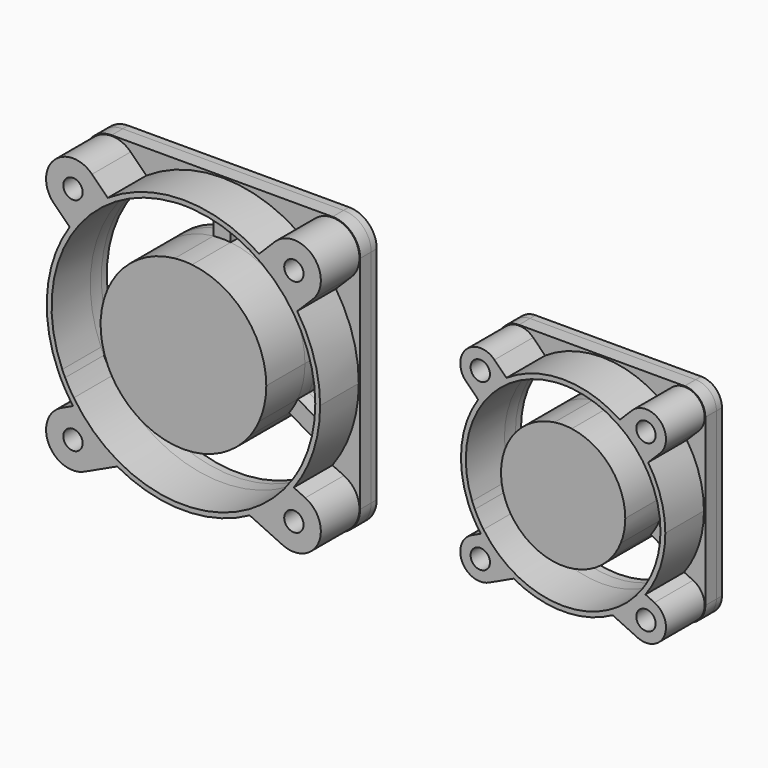
from build123d import *

# Parameters (mm, degrees)
F3_R     = 1.4
F4_DEPTH = 1
F5_DEPTH = 2
F6_DEPTH = 9
F7_DEPTH = 2
F8_DEPTH = 2


with BuildPart() as f4:
    # F3 (on Front) → F4 (new body)
    with BuildSketch(Plane.XZ):
        with BuildLine():
            Line((-16.757716, 18.757716), (-19.031282, 16.484151))
            ThreePointArc((-19.031282, 16.484151), (-15.999286, 14.000714), (-13.515849, 10.968718))
            Line((-13.515849, 10.968718), (-11.242284, 13.242284))
            ThreePointArc((-11.242284, 13.242284), (-11.242284, 18.757716), (-16.757716, 18.757716))
        make_face()
        with Locations((-14, 16)):
            Circle(F3_R, mode=Mode.SUBTRACT)
        with BuildLine():
            ThreePointArc((-45.981912, -11.688391), (-46.921843, -10.280624), (-47.738098, -8.79772))
            Line((-47.738098, -8.79772), (-50, -10.10363))
            Line((-50, -10.10363), (-50, -16))
            ThreePointArc((-50, -16), (-48.828427, -18.828427), (-46, -20))
            Line((-46, -20), (-30, -20))
            Line((-30, -20), (-14, -20))
            ThreePointArc((-14, -20), (-11.171573, -18.828427), (-10, -16))
            Line((-10, -16), (-10, 0))
            Line((-10, 0), (-10, 16))
            ThreePointArc((-10, 16), (-11.171573, 18.828427), (-14, 20))
            Line((-14, 20), (-30, 20))
            Line((-30, 20), (-46, 20))
            ThreePointArc((-46, 20), (-48.828427, 18.828427), (-50, 16))
            Line((-50, 16), (-50, 0))
            Line((-50, 0), (-50, -8.948929))
            Line((-50, -8.948929), (-48.16123, -7.887315))
            ThreePointArc((-48.16123, -7.887315), (-49.722147, 1.754112), (-46.484151, 10.968718))
            Line((-46.484151, 10.968718), (-48.757716, 13.242284))
            ThreePointArc((-48.757716, 13.242284), (-48.757716, 18.757716), (-43.242284, 18.757716))
            Line((-43.242284, 18.757716), (-40.968718, 16.484151))
            ThreePointArc((-40.968718, 16.484151), (-30, 19.8), (-19.031282, 16.484151))
            Line((-19.031282, 16.484151), (-16.757716, 18.757716))
            ThreePointArc((-16.757716, 18.757716), (-11.242284, 18.757716), (-11.242284, 13.242284))
            Line((-11.242284, 13.242284), (-13.515849, 10.968718))
            ThreePointArc((-13.515849, 10.968718), (-11.047082, 5.729477), (-10.2, 0))
            ThreePointArc((-10.2, 0), (-11.178711, -6.148095), (-14.018088, -11.688391))
            Line((-14.018088, -11.688391), (-12.351789, -12.4654))
            ThreePointArc((-12.351789, -12.4654), (-10.4654, -17.648211), (-15.648211, -19.5346))
            Line((-15.648211, -19.5346), (-20.401726, -17.318))
            ThreePointArc((-20.401726, -17.318), (-30, -19.8), (-39.598274, -17.318))
            Line((-39.598274, -17.318), (-44.351789, -19.5346))
            ThreePointArc((-44.351789, -19.5346), (-49.5346, -17.648211), (-47.648211, -12.4654))
            Line((-47.648211, -12.4654), (-45.981912, -11.688391))
        make_face()
        with BuildLine():
            ThreePointArc((-31.25, 19.059053), (-30, 19.1), (-28.75, 19.059053))
            ThreePointArc((-28.75, 19.059053), (-16.059322, 13.05632), (-10.9, 0))
            ThreePointArc((-10.9, 0), (-11.398859, -4.336766), (-12.869376, -8.446995))
            ThreePointArc((-12.869376, -8.446995), (-13.458915, -9.55), (-14.119376, -10.612058))
            ThreePointArc((-14.119376, -10.612058), (-30, -19.1), (-45.880624, -10.612058))
            ThreePointArc((-45.880624, -10.612058), (-46.541085, -9.55), (-47.130624, -8.446995))
            Line((-47.130624, -8.446995), (-47.738098, -8.79772))
            ThreePointArc((-47.738098, -8.79772), (-46.921843, -10.280624), (-45.981912, -11.688391))
            ThreePointArc((-45.981912, -11.688391), (-43.096168, -14.850266), (-39.598274, -17.318))
            ThreePointArc((-39.598274, -17.318), (-30, -19.8), (-20.401726, -17.318))
            ThreePointArc((-20.401726, -17.318), (-16.903832, -14.850266), (-14.018088, -11.688391))
            ThreePointArc((-14.018088, -11.688391), (-11.178711, -6.148095), (-10.2, 0))
            ThreePointArc((-10.2, 0), (-11.047082, 5.729477), (-13.515849, 10.968718))
            ThreePointArc((-13.515849, 10.968718), (-15.999286, 14.000714), (-19.031282, 16.484151))
            ThreePointArc((-19.031282, 16.484151), (-30, 19.8), (-40.968718, 16.484151))
            ThreePointArc((-40.968718, 16.484151), (-44.000714, 14.000714), (-46.484151, 10.968718))
            ThreePointArc((-46.484151, 10.968718), (-49.722147, 1.754112), (-48.16123, -7.887315))
            Line((-48.16123, -7.887315), (-47.550913, -7.534948))
            ThreePointArc((-47.550913, -7.534948), (-46.284312, 9.981542), (-31.25, 19.059053))
        make_face()
        with BuildLine():
            Line((-48.757716, 13.242284), (-46.484151, 10.968718))
            ThreePointArc((-46.484151, 10.968718), (-44.000714, 14.000714), (-40.968718, 16.484151))
            Line((-40.968718, 16.484151), (-43.242284, 18.757716))
            ThreePointArc((-43.242284, 18.757716), (-48.757716, 18.757716), (-48.757716, 13.242284))
        make_face()
        with Locations((-46, 16)):
            Circle(F3_R, mode=Mode.SUBTRACT)
        with BuildLine():
            ThreePointArc((-39.598274, -17.318), (-43.096168, -14.850266), (-45.981912, -11.688391))
            Line((-45.981912, -11.688391), (-47.648211, -12.4654))
            ThreePointArc((-47.648211, -12.4654), (-49.5346, -17.648211), (-44.351789, -19.5346))
            Line((-44.351789, -19.5346), (-39.598274, -17.318))
        make_face()
        with Locations((-46, -16)):
            Circle(F3_R, mode=Mode.SUBTRACT)
        with BuildLine():
            ThreePointArc((-14.018088, -11.688391), (-16.903832, -14.850266), (-20.401726, -17.318))
            Line((-20.401726, -17.318), (-15.648211, -19.5346))
            ThreePointArc((-15.648211, -19.5346), (-10.4654, -17.648211), (-12.351789, -12.4654))
            Line((-12.351789, -12.4654), (-14.018088, -11.688391))
        make_face()
        with Locations((-14, -16)):
            Circle(F3_R, mode=Mode.SUBTRACT)
        with BuildLine():
            Line((-12.869376, -8.446995), (-19.039231, -4.884827))
            ThreePointArc((-19.039231, -4.884827), (-19.607695, -6), (-20.289231, -7.049891))
            Line((-20.289231, -7.049891), (-14.119376, -10.612058))
            ThreePointArc((-14.119376, -10.612058), (-13.458915, -9.55), (-12.869376, -8.446995))
        make_face()
        with BuildLine():
            ThreePointArc((-39.710769, -7.049891), (-40.392305, -6), (-40.960769, -4.884827))
            Line((-40.960769, -4.884827), (-47.130624, -8.446995))
            ThreePointArc((-47.130624, -8.446995), (-46.541085, -9.55), (-45.880624, -10.612058))
            Line((-45.880624, -10.612058), (-39.710769, -7.049891))
        make_face()
        with BuildLine():
            ThreePointArc((-31.25, 11.934718), (-30, 12), (-28.75, 11.934718))
            Line((-28.75, 11.934718), (-28.75, 19.059053))
            ThreePointArc((-28.75, 19.059053), (-30, 19.1), (-31.25, 19.059053))
            Line((-31.25, 19.059053), (-31.25, 11.934718))
        make_face()
        with BuildLine():
            ThreePointArc((-28.75, 10.928746), (-21.791772, 7.322909), (-19, 0))
            ThreePointArc((-19, 0), (-19.230012, -2.237712), (-19.910428, -4.381841))
            Line((-19.910428, -4.381841), (-19.039231, -4.884827))
            ThreePointArc((-19.039231, -4.884827), (-18.262683, -2.497075), (-18, 0))
            ThreePointArc((-18, 0), (-21.083723, 8.031189), (-28.75, 11.934718))
            Line((-28.75, 11.934718), (-28.75, 10.928746))
        make_face()
        with BuildLine():
            Line((-19.039231, -4.884827), (-19.910428, -4.381841))
            ThreePointArc((-19.910428, -4.381841), (-20.473721, -5.5), (-21.160428, -6.546905))
            Line((-21.160428, -6.546905), (-20.289231, -7.049891))
            ThreePointArc((-20.289231, -7.049891), (-19.607695, -6), (-19.039231, -4.884827))
        make_face()
        with BuildLine():
            Line((-20.289231, -7.049891), (-21.160428, -6.546905))
            ThreePointArc((-21.160428, -6.546905), (-30, -11), (-38.839572, -6.546905))
            Line((-38.839572, -6.546905), (-39.710769, -7.049891))
            ThreePointArc((-39.710769, -7.049891), (-30, -12), (-20.289231, -7.049891))
        make_face()
        with BuildLine():
            ThreePointArc((-40.089572, -4.381841), (-39.526279, 5.5), (-31.25, 10.928746))
            Line((-31.25, 10.928746), (-31.25, 11.934718))
            ThreePointArc((-31.25, 11.934718), (-40.392305, 6), (-40.960769, -4.884827))
            Line((-40.960769, -4.884827), (-40.089572, -4.381841))
        make_face()
        with BuildLine():
            ThreePointArc((-38.839572, -6.546905), (-39.526279, -5.5), (-40.089572, -4.381841))
            Line((-40.089572, -4.381841), (-40.960769, -4.884827))
            ThreePointArc((-40.960769, -4.884827), (-40.392305, -6), (-39.710769, -7.049891))
            Line((-39.710769, -7.049891), (-38.839572, -6.546905))
        make_face()
        with BuildLine():
            ThreePointArc((-31.25, 10.928746), (-30, 11), (-28.75, 10.928746))
            Line((-28.75, 10.928746), (-28.75, 11.934718))
            ThreePointArc((-28.75, 11.934718), (-30, 12), (-31.25, 11.934718))
            Line((-31.25, 11.934718), (-31.25, 10.928746))
        make_face()
    extrude(amount=-F4_DEPTH)

    # F3 (on Front) → F5 (join)
    with BuildSketch(Plane.XZ):
        with BuildLine():
            ThreePointArc((-45.981912, -11.688391), (-46.921843, -10.280624), (-47.738098, -8.79772))
            Line((-47.738098, -8.79772), (-50, -10.10363))
            Line((-50, -10.10363), (-50, -16))
            ThreePointArc((-50, -16), (-48.828427, -18.828427), (-46, -20))
            Line((-46, -20), (-30, -20))
            Line((-30, -20), (-14, -20))
            ThreePointArc((-14, -20), (-11.171573, -18.828427), (-10, -16))
            Line((-10, -16), (-10, 0))
            Line((-10, 0), (-10, 16))
            ThreePointArc((-10, 16), (-11.171573, 18.828427), (-14, 20))
            Line((-14, 20), (-30, 20))
            Line((-30, 20), (-46, 20))
            ThreePointArc((-46, 20), (-48.828427, 18.828427), (-50, 16))
            Line((-50, 16), (-50, 0))
            Line((-50, 0), (-50, -8.948929))
            Line((-50, -8.948929), (-48.16123, -7.887315))
            ThreePointArc((-48.16123, -7.887315), (-49.722147, 1.754112), (-46.484151, 10.968718))
            Line((-46.484151, 10.968718), (-48.757716, 13.242284))
            ThreePointArc((-48.757716, 13.242284), (-48.757716, 18.757716), (-43.242284, 18.757716))
            Line((-43.242284, 18.757716), (-40.968718, 16.484151))
            ThreePointArc((-40.968718, 16.484151), (-30, 19.8), (-19.031282, 16.484151))
            Line((-19.031282, 16.484151), (-16.757716, 18.757716))
            ThreePointArc((-16.757716, 18.757716), (-11.242284, 18.757716), (-11.242284, 13.242284))
            Line((-11.242284, 13.242284), (-13.515849, 10.968718))
            ThreePointArc((-13.515849, 10.968718), (-11.047082, 5.729477), (-10.2, 0))
            ThreePointArc((-10.2, 0), (-11.178711, -6.148095), (-14.018088, -11.688391))
            Line((-14.018088, -11.688391), (-12.351789, -12.4654))
            ThreePointArc((-12.351789, -12.4654), (-10.4654, -17.648211), (-15.648211, -19.5346))
            Line((-15.648211, -19.5346), (-20.401726, -17.318))
            ThreePointArc((-20.401726, -17.318), (-30, -19.8), (-39.598274, -17.318))
            Line((-39.598274, -17.318), (-44.351789, -19.5346))
            ThreePointArc((-44.351789, -19.5346), (-49.5346, -17.648211), (-47.648211, -12.4654))
            Line((-47.648211, -12.4654), (-45.981912, -11.688391))
        make_face()
    extrude(amount=F5_DEPTH)

    # F3 (on Front) → F6, piece 2 (join)
    with BuildSketch(Plane.XZ):
        with BuildLine():
            Line((-16.757716, 18.757716), (-19.031282, 16.484151))
            ThreePointArc((-19.031282, 16.484151), (-15.999286, 14.000714), (-13.515849, 10.968718))
            Line((-13.515849, 10.968718), (-11.242284, 13.242284))
            ThreePointArc((-11.242284, 13.242284), (-11.242284, 18.757716), (-16.757716, 18.757716))
        make_face()
        with Locations((-14, 16)):
            Circle(F3_R, mode=Mode.SUBTRACT)
        with BuildLine():
            ThreePointArc((-14.018088, -11.688391), (-16.903832, -14.850266), (-20.401726, -17.318))
            Line((-20.401726, -17.318), (-15.648211, -19.5346))
            ThreePointArc((-15.648211, -19.5346), (-10.4654, -17.648211), (-12.351789, -12.4654))
            Line((-12.351789, -12.4654), (-14.018088, -11.688391))
        make_face()
        with Locations((-14, -16)):
            Circle(F3_R, mode=Mode.SUBTRACT)
        with BuildLine():
            ThreePointArc((-39.598274, -17.318), (-43.096168, -14.850266), (-45.981912, -11.688391))
            Line((-45.981912, -11.688391), (-47.648211, -12.4654))
            ThreePointArc((-47.648211, -12.4654), (-49.5346, -17.648211), (-44.351789, -19.5346))
            Line((-44.351789, -19.5346), (-39.598274, -17.318))
        make_face()
        with Locations((-46, -16)):
            Circle(F3_R, mode=Mode.SUBTRACT)
        with BuildLine():
            Line((-48.757716, 13.242284), (-46.484151, 10.968718))
            ThreePointArc((-46.484151, 10.968718), (-44.000714, 14.000714), (-40.968718, 16.484151))
            Line((-40.968718, 16.484151), (-43.242284, 18.757716))
            ThreePointArc((-43.242284, 18.757716), (-48.757716, 18.757716), (-48.757716, 13.242284))
        make_face()
        with Locations((-46, 16)):
            Circle(F3_R, mode=Mode.SUBTRACT)
        with BuildLine():
            ThreePointArc((-19.910428, -4.381841), (-19.230012, -2.237712), (-19, 0))
            ThreePointArc((-19, 0), (-21.791772, 7.322909), (-28.75, 10.928746))
            ThreePointArc((-28.75, 10.928746), (-30, 11), (-31.25, 10.928746))
            ThreePointArc((-31.25, 10.928746), (-39.526279, 5.5), (-40.089572, -4.381841))
            ThreePointArc((-40.089572, -4.381841), (-39.526279, -5.5), (-38.839572, -6.546905))
            ThreePointArc((-38.839572, -6.546905), (-30, -11), (-21.160428, -6.546905))
            ThreePointArc((-21.160428, -6.546905), (-20.473721, -5.5), (-19.910428, -4.381841))
        make_face()
        with BuildLine():
            ThreePointArc((-31.25, 19.059053), (-30, 19.1), (-28.75, 19.059053))
            ThreePointArc((-28.75, 19.059053), (-16.059322, 13.05632), (-10.9, 0))
            ThreePointArc((-10.9, 0), (-11.398859, -4.336766), (-12.869376, -8.446995))
            ThreePointArc((-12.869376, -8.446995), (-13.458915, -9.55), (-14.119376, -10.612058))
            ThreePointArc((-14.119376, -10.612058), (-30, -19.1), (-45.880624, -10.612058))
            ThreePointArc((-45.880624, -10.612058), (-46.541085, -9.55), (-47.130624, -8.446995))
            Line((-47.130624, -8.446995), (-47.738098, -8.79772))
            ThreePointArc((-47.738098, -8.79772), (-46.921843, -10.280624), (-45.981912, -11.688391))
            ThreePointArc((-45.981912, -11.688391), (-43.096168, -14.850266), (-39.598274, -17.318))
            ThreePointArc((-39.598274, -17.318), (-30, -19.8), (-20.401726, -17.318))
            ThreePointArc((-20.401726, -17.318), (-16.903832, -14.850266), (-14.018088, -11.688391))
            ThreePointArc((-14.018088, -11.688391), (-11.178711, -6.148095), (-10.2, 0))
            ThreePointArc((-10.2, 0), (-11.047082, 5.729477), (-13.515849, 10.968718))
            ThreePointArc((-13.515849, 10.968718), (-15.999286, 14.000714), (-19.031282, 16.484151))
            ThreePointArc((-19.031282, 16.484151), (-30, 19.8), (-40.968718, 16.484151))
            ThreePointArc((-40.968718, 16.484151), (-44.000714, 14.000714), (-46.484151, 10.968718))
            ThreePointArc((-46.484151, 10.968718), (-49.722147, 1.754112), (-48.16123, -7.887315))
            Line((-48.16123, -7.887315), (-47.550913, -7.534948))
            ThreePointArc((-47.550913, -7.534948), (-46.284312, 9.981542), (-31.25, 19.059053))
        make_face()
        with BuildLine():
            ThreePointArc((-28.75, 10.928746), (-21.791772, 7.322909), (-19, 0))
            ThreePointArc((-19, 0), (-19.230012, -2.237712), (-19.910428, -4.381841))
            Line((-19.910428, -4.381841), (-19.039231, -4.884827))
            ThreePointArc((-19.039231, -4.884827), (-18.262683, -2.497075), (-18, 0))
            ThreePointArc((-18, 0), (-21.083723, 8.031189), (-28.75, 11.934718))
            Line((-28.75, 11.934718), (-28.75, 10.928746))
        make_face()
        with BuildLine():
            ThreePointArc((-31.25, 10.928746), (-30, 11), (-28.75, 10.928746))
            Line((-28.75, 10.928746), (-28.75, 11.934718))
            ThreePointArc((-28.75, 11.934718), (-30, 12), (-31.25, 11.934718))
            Line((-31.25, 11.934718), (-31.25, 10.928746))
        make_face()
        with BuildLine():
            ThreePointArc((-40.089572, -4.381841), (-39.526279, 5.5), (-31.25, 10.928746))
            Line((-31.25, 10.928746), (-31.25, 11.934718))
            ThreePointArc((-31.25, 11.934718), (-40.392305, 6), (-40.960769, -4.884827))
            Line((-40.960769, -4.884827), (-40.089572, -4.381841))
        make_face()
        with BuildLine():
            ThreePointArc((-38.839572, -6.546905), (-39.526279, -5.5), (-40.089572, -4.381841))
            Line((-40.089572, -4.381841), (-40.960769, -4.884827))
            ThreePointArc((-40.960769, -4.884827), (-40.392305, -6), (-39.710769, -7.049891))
            Line((-39.710769, -7.049891), (-38.839572, -6.546905))
        make_face()
        with BuildLine():
            Line((-20.289231, -7.049891), (-21.160428, -6.546905))
            ThreePointArc((-21.160428, -6.546905), (-30, -11), (-38.839572, -6.546905))
            Line((-38.839572, -6.546905), (-39.710769, -7.049891))
            ThreePointArc((-39.710769, -7.049891), (-30, -12), (-20.289231, -7.049891))
        make_face()
        with BuildLine():
            Line((-19.039231, -4.884827), (-19.910428, -4.381841))
            ThreePointArc((-19.910428, -4.381841), (-20.473721, -5.5), (-21.160428, -6.546905))
            Line((-21.160428, -6.546905), (-20.289231, -7.049891))
            ThreePointArc((-20.289231, -7.049891), (-19.607695, -6), (-19.039231, -4.884827))
        make_face()
        with BuildLine():
            Line((-47.738098, -8.79772), (-47.130624, -8.446995))
            ThreePointArc((-47.130624, -8.446995), (-47.346764, -7.993734), (-47.550913, -7.534948))
            Line((-47.550913, -7.534948), (-48.16123, -7.887315))
            ThreePointArc((-48.16123, -7.887315), (-47.955435, -8.3452), (-47.738098, -8.79772))
        make_face()
    extrude(amount=F6_DEPTH)


with BuildPart() as f4b:
    # F3 (on Front) → F4, piece 2 (new body)
    with BuildSketch(Plane.XZ):
        with BuildLine():
            ThreePointArc((36.925159, -8.765305), (34.773744, -11.113682), (32.169719, -12.947399))
            Line((32.169719, -12.947399), (35.774407, -14.628293))
            ThreePointArc((35.774407, -14.628293), (39.628293, -13.225593), (38.225593, -9.371707))
            Line((38.225593, -9.371707), (36.925159, -8.765305))
        make_face()
        with Locations((37, -12)):
            Circle(F3_R, mode=Mode.SUBTRACT)
        with BuildLine():
            ThreePointArc((13.074841, -8.765305), (12.278931, -7.564021), (11.603621, -6.291027))
            Line((11.603621, -6.291027), (10, -7.216878))
            Line((10, -7.216878), (10, -12))
            ThreePointArc((10, -12), (10.87868, -14.12132), (13, -15))
            Line((13, -15), (25, -15))
            Line((25, -15), (37, -15))
            ThreePointArc((37, -15), (39.12132, -14.12132), (40, -12))
            Line((40, -12), (40, 0))
            Line((40, 0), (40, 12))
            ThreePointArc((40, 12), (39.12132, 14.12132), (37, 15))
            Line((37, 15), (25, 15))
            Line((25, 15), (13, 15))
            ThreePointArc((13, 15), (10.87868, 14.12132), (10, 12))
            Line((10, 12), (10, 0))
            Line((10, 0), (10, -6.062178))
            Line((10, -6.062178), (11.206807, -5.365428))
            ThreePointArc((11.206807, -5.365428), (10.287187, 1.604095), (12.687081, 8.2117))
            Line((12.687081, 8.2117), (10.94939, 9.94939))
            ThreePointArc((10.94939, 9.94939), (10.94939, 14.05061), (15.05061, 14.05061))
            Line((15.05061, 14.05061), (16.7883, 12.312919))
            ThreePointArc((16.7883, 12.312919), (25, 14.8), (33.2117, 12.312919))
            Line((33.2117, 12.312919), (34.94939, 14.05061))
            ThreePointArc((34.94939, 14.05061), (39.05061, 14.05061), (39.05061, 9.94939))
            Line((39.05061, 9.94939), (37.312919, 8.2117))
            ThreePointArc((37.312919, 8.2117), (39.16459, 4.290035), (39.8, 0))
            ThreePointArc((39.8, 0), (39.062936, -4.612355), (36.925159, -8.765305))
            Line((36.925159, -8.765305), (38.225593, -9.371707))
            ThreePointArc((38.225593, -9.371707), (39.628293, -13.225593), (35.774407, -14.628293))
            Line((35.774407, -14.628293), (32.169719, -12.947399))
            ThreePointArc((32.169719, -12.947399), (25, -14.8), (17.830281, -12.947399))
            Line((17.830281, -12.947399), (14.225593, -14.628293))
            ThreePointArc((14.225593, -14.628293), (10.371707, -13.225593), (11.774407, -9.371707))
            Line((11.774407, -9.371707), (13.074841, -8.765305))
        make_face()
        with BuildLine():
            ThreePointArc((17.830281, -12.947399), (15.226256, -11.113682), (13.074841, -8.765305))
            Line((13.074841, -8.765305), (11.774407, -9.371707))
            ThreePointArc((11.774407, -9.371707), (10.371707, -13.225593), (14.225593, -14.628293))
            Line((14.225593, -14.628293), (17.830281, -12.947399))
        make_face()
        with Locations((13, -12)):
            Circle(F3_R, mode=Mode.SUBTRACT)
        with BuildLine():
            Line((10.94939, 9.94939), (12.687081, 8.2117))
            ThreePointArc((12.687081, 8.2117), (14.53482, 10.46518), (16.7883, 12.312919))
            Line((16.7883, 12.312919), (15.05061, 14.05061))
            ThreePointArc((15.05061, 14.05061), (10.94939, 14.05061), (10.94939, 9.94939))
        make_face()
        with Locations((13, 12)):
            Circle(F3_R, mode=Mode.SUBTRACT)
        with BuildLine():
            Line((34.94939, 14.05061), (33.2117, 12.312919))
            ThreePointArc((33.2117, 12.312919), (35.46518, 10.46518), (37.312919, 8.2117))
            Line((37.312919, 8.2117), (39.05061, 9.94939))
            ThreePointArc((39.05061, 9.94939), (39.05061, 14.05061), (34.94939, 14.05061))
        make_face()
        with Locations((37, 12)):
            Circle(F3_R, mode=Mode.SUBTRACT)
        with BuildLine():
            ThreePointArc((23.75, 14.044483), (25, 14.1), (26.25, 14.044483))
            ThreePointArc((26.25, 14.044483), (35.402764, 9.518009), (39.1, 0))
            ThreePointArc((39.1, 0), (38.768063, -3.041456), (37.787879, -5.93971))
            ThreePointArc((37.787879, -5.93971), (37.210958, -7.05), (36.537879, -8.104773))
            ThreePointArc((36.537879, -8.104773), (25, -14.1), (13.462121, -8.104773))
            ThreePointArc((13.462121, -8.104773), (12.789042, -7.05), (12.212121, -5.93971))
            Line((12.212121, -5.93971), (11.603621, -6.291027))
            ThreePointArc((11.603621, -6.291027), (12.278931, -7.564021), (13.074841, -8.765305))
            ThreePointArc((13.074841, -8.765305), (15.226256, -11.113682), (17.830281, -12.947399))
            ThreePointArc((17.830281, -12.947399), (25, -14.8), (32.169719, -12.947399))
            ThreePointArc((32.169719, -12.947399), (34.773744, -11.113682), (36.925159, -8.765305))
            ThreePointArc((36.925159, -8.765305), (39.062936, -4.612355), (39.8, 0))
            ThreePointArc((39.8, 0), (39.16459, 4.290035), (37.312919, 8.2117))
            ThreePointArc((37.312919, 8.2117), (35.46518, 10.46518), (33.2117, 12.312919))
            ThreePointArc((33.2117, 12.312919), (25, 14.8), (16.7883, 12.312919))
            ThreePointArc((16.7883, 12.312919), (14.53482, 10.46518), (12.687081, 8.2117))
            ThreePointArc((12.687081, 8.2117), (10.287187, 1.604095), (11.206807, -5.365428))
            Line((11.206807, -5.365428), (11.820514, -5.011103))
            ThreePointArc((11.820514, -5.011103), (13.048793, 7.481888), (23.75, 14.044483))
        make_face()
        with BuildLine():
            Line((37.787879, -5.93971), (33.343687, -3.373854))
            ThreePointArc((33.343687, -3.373854), (32.794229, -4.5), (32.093687, -5.538918))
            Line((32.093687, -5.538918), (36.537879, -8.104773))
            ThreePointArc((36.537879, -8.104773), (37.210958, -7.05), (37.787879, -5.93971))
        make_face()
        with BuildLine():
            ThreePointArc((17.906313, -5.538918), (17.205771, -4.5), (16.656313, -3.373854))
            Line((16.656313, -3.373854), (12.212121, -5.93971))
            ThreePointArc((12.212121, -5.93971), (12.789042, -7.05), (13.462121, -8.104773))
            Line((13.462121, -8.104773), (17.906313, -5.538918))
        make_face()
        with BuildLine():
            ThreePointArc((26.25, 8.154753), (31.259992, 5.373546), (33.25, 0))
            ThreePointArc((33.25, 0), (33.108085, -1.523632), (32.687223, -2.994845))
            Line((32.687223, -2.994845), (33.343687, -3.373854))
            ThreePointArc((33.343687, -3.373854), (33.834398, -1.718549), (34, 0))
            ThreePointArc((34, 0), (31.791539, 5.905506), (26.25, 8.912772))
            Line((26.25, 8.912772), (26.25, 8.154753))
        make_face()
        with BuildLine():
            Line((33.343687, -3.373854), (32.687223, -2.994845))
            ThreePointArc((32.687223, -2.994845), (32.14471, -4.125), (31.437223, -5.159908))
            Line((31.437223, -5.159908), (32.093687, -5.538918))
            ThreePointArc((32.093687, -5.538918), (32.794229, -4.5), (33.343687, -3.373854))
        make_face()
        with BuildLine():
            Line((32.093687, -5.538918), (31.437223, -5.159908))
            ThreePointArc((31.437223, -5.159908), (25, -8.25), (18.562777, -5.159908))
            Line((18.562777, -5.159908), (17.906313, -5.538918))
            ThreePointArc((17.906313, -5.538918), (25, -9), (32.093687, -5.538918))
        make_face()
        with BuildLine():
            ThreePointArc((17.312777, -2.994845), (17.85529, 4.125), (23.75, 8.154753))
            Line((23.75, 8.154753), (23.75, 8.912772))
            ThreePointArc((23.75, 8.912772), (17.205771, 4.5), (16.656313, -3.373854))
            Line((16.656313, -3.373854), (17.312777, -2.994845))
        make_face()
        with BuildLine():
            ThreePointArc((18.562777, -5.159908), (17.85529, -4.125), (17.312777, -2.994845))
            Line((17.312777, -2.994845), (16.656313, -3.373854))
            ThreePointArc((16.656313, -3.373854), (17.205771, -4.5), (17.906313, -5.538918))
            Line((17.906313, -5.538918), (18.562777, -5.159908))
        make_face()
        with BuildLine():
            ThreePointArc((23.75, 8.154753), (25, 8.25), (26.25, 8.154753))
            Line((26.25, 8.154753), (26.25, 8.912772))
            ThreePointArc((26.25, 8.912772), (25, 9), (23.75, 8.912772))
            Line((23.75, 8.912772), (23.75, 8.154753))
        make_face()
        with BuildLine():
            ThreePointArc((23.75, 8.912772), (25, 9), (26.25, 8.912772))
            Line((26.25, 8.912772), (26.25, 14.044483))
            ThreePointArc((26.25, 14.044483), (25, 14.1), (23.75, 14.044483))
            Line((23.75, 14.044483), (23.75, 8.912772))
        make_face()
    extrude(amount=-F4_DEPTH)

    # F3 (on Front) → F5, piece 2 (join)
    with BuildSketch(Plane.XZ):
        with BuildLine():
            ThreePointArc((13.074841, -8.765305), (12.278931, -7.564021), (11.603621, -6.291027))
            Line((11.603621, -6.291027), (10, -7.216878))
            Line((10, -7.216878), (10, -12))
            ThreePointArc((10, -12), (10.87868, -14.12132), (13, -15))
            Line((13, -15), (25, -15))
            Line((25, -15), (37, -15))
            ThreePointArc((37, -15), (39.12132, -14.12132), (40, -12))
            Line((40, -12), (40, 0))
            Line((40, 0), (40, 12))
            ThreePointArc((40, 12), (39.12132, 14.12132), (37, 15))
            Line((37, 15), (25, 15))
            Line((25, 15), (13, 15))
            ThreePointArc((13, 15), (10.87868, 14.12132), (10, 12))
            Line((10, 12), (10, 0))
            Line((10, 0), (10, -6.062178))
            Line((10, -6.062178), (11.206807, -5.365428))
            ThreePointArc((11.206807, -5.365428), (10.287187, 1.604095), (12.687081, 8.2117))
            Line((12.687081, 8.2117), (10.94939, 9.94939))
            ThreePointArc((10.94939, 9.94939), (10.94939, 14.05061), (15.05061, 14.05061))
            Line((15.05061, 14.05061), (16.7883, 12.312919))
            ThreePointArc((16.7883, 12.312919), (25, 14.8), (33.2117, 12.312919))
            Line((33.2117, 12.312919), (34.94939, 14.05061))
            ThreePointArc((34.94939, 14.05061), (39.05061, 14.05061), (39.05061, 9.94939))
            Line((39.05061, 9.94939), (37.312919, 8.2117))
            ThreePointArc((37.312919, 8.2117), (39.16459, 4.290035), (39.8, 0))
            ThreePointArc((39.8, 0), (39.062936, -4.612355), (36.925159, -8.765305))
            Line((36.925159, -8.765305), (38.225593, -9.371707))
            ThreePointArc((38.225593, -9.371707), (39.628293, -13.225593), (35.774407, -14.628293))
            Line((35.774407, -14.628293), (32.169719, -12.947399))
            ThreePointArc((32.169719, -12.947399), (25, -14.8), (17.830281, -12.947399))
            Line((17.830281, -12.947399), (14.225593, -14.628293))
            ThreePointArc((14.225593, -14.628293), (10.371707, -13.225593), (11.774407, -9.371707))
            Line((11.774407, -9.371707), (13.074841, -8.765305))
        make_face()
    extrude(amount=F5_DEPTH)

    # F3 (on Front) → F6 (join)
    with BuildSketch(Plane.XZ):
        with BuildLine():
            ThreePointArc((23.75, 14.044483), (25, 14.1), (26.25, 14.044483))
            ThreePointArc((26.25, 14.044483), (35.402764, 9.518009), (39.1, 0))
            ThreePointArc((39.1, 0), (38.768063, -3.041456), (37.787879, -5.93971))
            ThreePointArc((37.787879, -5.93971), (37.210958, -7.05), (36.537879, -8.104773))
            ThreePointArc((36.537879, -8.104773), (25, -14.1), (13.462121, -8.104773))
            ThreePointArc((13.462121, -8.104773), (12.789042, -7.05), (12.212121, -5.93971))
            Line((12.212121, -5.93971), (11.603621, -6.291027))
            ThreePointArc((11.603621, -6.291027), (12.278931, -7.564021), (13.074841, -8.765305))
            ThreePointArc((13.074841, -8.765305), (15.226256, -11.113682), (17.830281, -12.947399))
            ThreePointArc((17.830281, -12.947399), (25, -14.8), (32.169719, -12.947399))
            ThreePointArc((32.169719, -12.947399), (34.773744, -11.113682), (36.925159, -8.765305))
            ThreePointArc((36.925159, -8.765305), (39.062936, -4.612355), (39.8, 0))
            ThreePointArc((39.8, 0), (39.16459, 4.290035), (37.312919, 8.2117))
            ThreePointArc((37.312919, 8.2117), (35.46518, 10.46518), (33.2117, 12.312919))
            ThreePointArc((33.2117, 12.312919), (25, 14.8), (16.7883, 12.312919))
            ThreePointArc((16.7883, 12.312919), (14.53482, 10.46518), (12.687081, 8.2117))
            ThreePointArc((12.687081, 8.2117), (10.287187, 1.604095), (11.206807, -5.365428))
            Line((11.206807, -5.365428), (11.820514, -5.011103))
            ThreePointArc((11.820514, -5.011103), (13.048793, 7.481888), (23.75, 14.044483))
        make_face()
        with BuildLine():
            Line((34.94939, 14.05061), (33.2117, 12.312919))
            ThreePointArc((33.2117, 12.312919), (35.46518, 10.46518), (37.312919, 8.2117))
            Line((37.312919, 8.2117), (39.05061, 9.94939))
            ThreePointArc((39.05061, 9.94939), (39.05061, 14.05061), (34.94939, 14.05061))
        make_face()
        with Locations((37, 12)):
            Circle(F3_R, mode=Mode.SUBTRACT)
        with BuildLine():
            Line((11.603621, -6.291027), (12.212121, -5.93971))
            ThreePointArc((12.212121, -5.93971), (12.008018, -5.478906), (11.820514, -5.011103))
            Line((11.820514, -5.011103), (11.206807, -5.365428))
            ThreePointArc((11.206807, -5.365428), (11.397339, -5.831604), (11.603621, -6.291027))
        make_face()
        with BuildLine():
            ThreePointArc((32.687223, -2.994845), (33.108085, -1.523632), (33.25, 0))
            ThreePointArc((33.25, 0), (31.259992, 5.373546), (26.25, 8.154753))
            ThreePointArc((26.25, 8.154753), (25, 8.25), (23.75, 8.154753))
            ThreePointArc((23.75, 8.154753), (17.85529, 4.125), (17.312777, -2.994845))
            ThreePointArc((17.312777, -2.994845), (17.85529, -4.125), (18.562777, -5.159908))
            ThreePointArc((18.562777, -5.159908), (25, -8.25), (31.437223, -5.159908))
            ThreePointArc((31.437223, -5.159908), (32.14471, -4.125), (32.687223, -2.994845))
        make_face()
        with BuildLine():
            ThreePointArc((17.312777, -2.994845), (17.85529, 4.125), (23.75, 8.154753))
            Line((23.75, 8.154753), (23.75, 8.912772))
            ThreePointArc((23.75, 8.912772), (17.205771, 4.5), (16.656313, -3.373854))
            Line((16.656313, -3.373854), (17.312777, -2.994845))
        make_face()
        with BuildLine():
            ThreePointArc((26.25, 8.154753), (31.259992, 5.373546), (33.25, 0))
            ThreePointArc((33.25, 0), (33.108085, -1.523632), (32.687223, -2.994845))
            Line((32.687223, -2.994845), (33.343687, -3.373854))
            ThreePointArc((33.343687, -3.373854), (33.834398, -1.718549), (34, 0))
            ThreePointArc((34, 0), (31.791539, 5.905506), (26.25, 8.912772))
            Line((26.25, 8.912772), (26.25, 8.154753))
        make_face()
        with BuildLine():
            ThreePointArc((23.75, 8.154753), (25, 8.25), (26.25, 8.154753))
            Line((26.25, 8.154753), (26.25, 8.912772))
            ThreePointArc((26.25, 8.912772), (25, 9), (23.75, 8.912772))
            Line((23.75, 8.912772), (23.75, 8.154753))
        make_face()
        with BuildLine():
            Line((33.343687, -3.373854), (32.687223, -2.994845))
            ThreePointArc((32.687223, -2.994845), (32.14471, -4.125), (31.437223, -5.159908))
            Line((31.437223, -5.159908), (32.093687, -5.538918))
            ThreePointArc((32.093687, -5.538918), (32.794229, -4.5), (33.343687, -3.373854))
        make_face()
        with BuildLine():
            ThreePointArc((18.562777, -5.159908), (17.85529, -4.125), (17.312777, -2.994845))
            Line((17.312777, -2.994845), (16.656313, -3.373854))
            ThreePointArc((16.656313, -3.373854), (17.205771, -4.5), (17.906313, -5.538918))
            Line((17.906313, -5.538918), (18.562777, -5.159908))
        make_face()
        with BuildLine():
            Line((32.093687, -5.538918), (31.437223, -5.159908))
            ThreePointArc((31.437223, -5.159908), (25, -8.25), (18.562777, -5.159908))
            Line((18.562777, -5.159908), (17.906313, -5.538918))
            ThreePointArc((17.906313, -5.538918), (25, -9), (32.093687, -5.538918))
        make_face()
        with BuildLine():
            ThreePointArc((36.925159, -8.765305), (34.773744, -11.113682), (32.169719, -12.947399))
            Line((32.169719, -12.947399), (35.774407, -14.628293))
            ThreePointArc((35.774407, -14.628293), (39.628293, -13.225593), (38.225593, -9.371707))
            Line((38.225593, -9.371707), (36.925159, -8.765305))
        make_face()
        with Locations((37, -12)):
            Circle(F3_R, mode=Mode.SUBTRACT)
        with BuildLine():
            ThreePointArc((17.830281, -12.947399), (15.226256, -11.113682), (13.074841, -8.765305))
            Line((13.074841, -8.765305), (11.774407, -9.371707))
            ThreePointArc((11.774407, -9.371707), (10.371707, -13.225593), (14.225593, -14.628293))
            Line((14.225593, -14.628293), (17.830281, -12.947399))
        make_face()
        with Locations((13, -12)):
            Circle(F3_R, mode=Mode.SUBTRACT)
        with BuildLine():
            Line((10.94939, 9.94939), (12.687081, 8.2117))
            ThreePointArc((12.687081, 8.2117), (14.53482, 10.46518), (16.7883, 12.312919))
            Line((16.7883, 12.312919), (15.05061, 14.05061))
            ThreePointArc((15.05061, 14.05061), (10.94939, 14.05061), (10.94939, 9.94939))
        make_face()
        with Locations((13, 12)):
            Circle(F3_R, mode=Mode.SUBTRACT)
    extrude(amount=F6_DEPTH)


with BuildPart() as f7_tool:
    # F3 (on Front) → F7 (new body)
    with BuildSketch(Plane.XZ):
        with BuildLine():
            Line((11.603621, -6.291027), (12.212121, -5.93971))
            ThreePointArc((12.212121, -5.93971), (12.008018, -5.478906), (11.820514, -5.011103))
            Line((11.820514, -5.011103), (11.206807, -5.365428))
            ThreePointArc((11.206807, -5.365428), (11.397339, -5.831604), (11.603621, -6.291027))
        make_face()
        with BuildLine():
            Line((-47.738098, -8.79772), (-47.130624, -8.446995))
            ThreePointArc((-47.130624, -8.446995), (-47.346764, -7.993734), (-47.550913, -7.534948))
            Line((-47.550913, -7.534948), (-48.16123, -7.887315))
            ThreePointArc((-48.16123, -7.887315), (-47.955435, -8.3452), (-47.738098, -8.79772))
        make_face()
    extrude(amount=F7_DEPTH)


with BuildPart() as f4_1:
    add(f4.part)

    # F7: cut by f7_tool
    add(f7_tool.part, mode=Mode.SUBTRACT)


with BuildPart() as f4b_1:
    add(f4b.part)

    # F7: cut by f7_tool
    add(f7_tool.part, mode=Mode.SUBTRACT)


with BuildPart() as f8:
    # F3 (on Front) → F8 (new body)
    with BuildSketch(Plane.XZ):
        with BuildLine():
            ThreePointArc((-45.981912, -11.688391), (-46.921843, -10.280624), (-47.738098, -8.79772))
            Line((-47.738098, -8.79772), (-50, -10.10363))
            Line((-50, -10.10363), (-50, -16))
            ThreePointArc((-50, -16), (-48.828427, -18.828427), (-46, -20))
            Line((-46, -20), (-30, -20))
            Line((-30, -20), (-14, -20))
            ThreePointArc((-14, -20), (-11.171573, -18.828427), (-10, -16))
            Line((-10, -16), (-10, 0))
            Line((-10, 0), (-10, 16))
            ThreePointArc((-10, 16), (-11.171573, 18.828427), (-14, 20))
            Line((-14, 20), (-30, 20))
            Line((-30, 20), (-46, 20))
            ThreePointArc((-46, 20), (-48.828427, 18.828427), (-50, 16))
            Line((-50, 16), (-50, 0))
            Line((-50, 0), (-50, -8.948929))
            Line((-50, -8.948929), (-48.16123, -7.887315))
            ThreePointArc((-48.16123, -7.887315), (-49.722147, 1.754112), (-46.484151, 10.968718))
            Line((-46.484151, 10.968718), (-48.757716, 13.242284))
            ThreePointArc((-48.757716, 13.242284), (-48.757716, 18.757716), (-43.242284, 18.757716))
            Line((-43.242284, 18.757716), (-40.968718, 16.484151))
            ThreePointArc((-40.968718, 16.484151), (-30, 19.8), (-19.031282, 16.484151))
            Line((-19.031282, 16.484151), (-16.757716, 18.757716))
            ThreePointArc((-16.757716, 18.757716), (-11.242284, 18.757716), (-11.242284, 13.242284))
            Line((-11.242284, 13.242284), (-13.515849, 10.968718))
            ThreePointArc((-13.515849, 10.968718), (-11.047082, 5.729477), (-10.2, 0))
            ThreePointArc((-10.2, 0), (-11.178711, -6.148095), (-14.018088, -11.688391))
            Line((-14.018088, -11.688391), (-12.351789, -12.4654))
            ThreePointArc((-12.351789, -12.4654), (-10.4654, -17.648211), (-15.648211, -19.5346))
            Line((-15.648211, -19.5346), (-20.401726, -17.318))
            ThreePointArc((-20.401726, -17.318), (-30, -19.8), (-39.598274, -17.318))
            Line((-39.598274, -17.318), (-44.351789, -19.5346))
            ThreePointArc((-44.351789, -19.5346), (-49.5346, -17.648211), (-47.648211, -12.4654))
            Line((-47.648211, -12.4654), (-45.981912, -11.688391))
        make_face()
        with BuildLine():
            Line((-16.757716, 18.757716), (-19.031282, 16.484151))
            ThreePointArc((-19.031282, 16.484151), (-15.999286, 14.000714), (-13.515849, 10.968718))
            Line((-13.515849, 10.968718), (-11.242284, 13.242284))
            ThreePointArc((-11.242284, 13.242284), (-11.242284, 18.757716), (-16.757716, 18.757716))
        make_face()
        with Locations((-14, 16)):
            Circle(F3_R, mode=Mode.SUBTRACT)
        with BuildLine():
            Line((-48.757716, 13.242284), (-46.484151, 10.968718))
            ThreePointArc((-46.484151, 10.968718), (-44.000714, 14.000714), (-40.968718, 16.484151))
            Line((-40.968718, 16.484151), (-43.242284, 18.757716))
            ThreePointArc((-43.242284, 18.757716), (-48.757716, 18.757716), (-48.757716, 13.242284))
        make_face()
        with Locations((-46, 16)):
            Circle(F3_R, mode=Mode.SUBTRACT)
        with BuildLine():
            ThreePointArc((-39.598274, -17.318), (-43.096168, -14.850266), (-45.981912, -11.688391))
            Line((-45.981912, -11.688391), (-47.648211, -12.4654))
            ThreePointArc((-47.648211, -12.4654), (-49.5346, -17.648211), (-44.351789, -19.5346))
            Line((-44.351789, -19.5346), (-39.598274, -17.318))
        make_face()
        with Locations((-46, -16)):
            Circle(F3_R, mode=Mode.SUBTRACT)
        with BuildLine():
            ThreePointArc((-14.018088, -11.688391), (-16.903832, -14.850266), (-20.401726, -17.318))
            Line((-20.401726, -17.318), (-15.648211, -19.5346))
            ThreePointArc((-15.648211, -19.5346), (-10.4654, -17.648211), (-12.351789, -12.4654))
            Line((-12.351789, -12.4654), (-14.018088, -11.688391))
        make_face()
        with Locations((-14, -16)):
            Circle(F3_R, mode=Mode.SUBTRACT)
        with BuildLine():
            Line((-12.869376, -8.446995), (-19.039231, -4.884827))
            ThreePointArc((-19.039231, -4.884827), (-19.607695, -6), (-20.289231, -7.049891))
            Line((-20.289231, -7.049891), (-14.119376, -10.612058))
            ThreePointArc((-14.119376, -10.612058), (-13.458915, -9.55), (-12.869376, -8.446995))
        make_face()
        with BuildLine():
            ThreePointArc((-19.910428, -4.381841), (-19.230012, -2.237712), (-19, 0))
            ThreePointArc((-19, 0), (-21.791772, 7.322909), (-28.75, 10.928746))
            ThreePointArc((-28.75, 10.928746), (-30, 11), (-31.25, 10.928746))
            ThreePointArc((-31.25, 10.928746), (-39.526279, 5.5), (-40.089572, -4.381841))
            ThreePointArc((-40.089572, -4.381841), (-39.526279, -5.5), (-38.839572, -6.546905))
            ThreePointArc((-38.839572, -6.546905), (-30, -11), (-21.160428, -6.546905))
            ThreePointArc((-21.160428, -6.546905), (-20.473721, -5.5), (-19.910428, -4.381841))
        make_face()
        with BuildLine():
            ThreePointArc((-31.25, 11.934718), (-30, 12), (-28.75, 11.934718))
            Line((-28.75, 11.934718), (-28.75, 19.059053))
            ThreePointArc((-28.75, 19.059053), (-30, 19.1), (-31.25, 19.059053))
            Line((-31.25, 19.059053), (-31.25, 11.934718))
        make_face()
        with BuildLine():
            ThreePointArc((-39.710769, -7.049891), (-40.392305, -6), (-40.960769, -4.884827))
            Line((-40.960769, -4.884827), (-47.130624, -8.446995))
            ThreePointArc((-47.130624, -8.446995), (-46.541085, -9.55), (-45.880624, -10.612058))
            Line((-45.880624, -10.612058), (-39.710769, -7.049891))
        make_face()
        with BuildLine():
            Line((-50, -10.10363), (-47.738098, -8.79772))
            ThreePointArc((-47.738098, -8.79772), (-47.955435, -8.3452), (-48.16123, -7.887315))
            Line((-48.16123, -7.887315), (-50, -8.948929))
            Line((-50, -8.948929), (-50, -10.10363))
        make_face()
        with BuildLine():
            ThreePointArc((-31.25, 19.059053), (-30, 19.1), (-28.75, 19.059053))
            ThreePointArc((-28.75, 19.059053), (-16.059322, 13.05632), (-10.9, 0))
            ThreePointArc((-10.9, 0), (-11.398859, -4.336766), (-12.869376, -8.446995))
            ThreePointArc((-12.869376, -8.446995), (-13.458915, -9.55), (-14.119376, -10.612058))
            ThreePointArc((-14.119376, -10.612058), (-30, -19.1), (-45.880624, -10.612058))
            ThreePointArc((-45.880624, -10.612058), (-46.541085, -9.55), (-47.130624, -8.446995))
            Line((-47.130624, -8.446995), (-47.738098, -8.79772))
            ThreePointArc((-47.738098, -8.79772), (-46.921843, -10.280624), (-45.981912, -11.688391))
            ThreePointArc((-45.981912, -11.688391), (-43.096168, -14.850266), (-39.598274, -17.318))
            ThreePointArc((-39.598274, -17.318), (-30, -19.8), (-20.401726, -17.318))
            ThreePointArc((-20.401726, -17.318), (-16.903832, -14.850266), (-14.018088, -11.688391))
            ThreePointArc((-14.018088, -11.688391), (-11.178711, -6.148095), (-10.2, 0))
            ThreePointArc((-10.2, 0), (-11.047082, 5.729477), (-13.515849, 10.968718))
            ThreePointArc((-13.515849, 10.968718), (-15.999286, 14.000714), (-19.031282, 16.484151))
            ThreePointArc((-19.031282, 16.484151), (-30, 19.8), (-40.968718, 16.484151))
            ThreePointArc((-40.968718, 16.484151), (-44.000714, 14.000714), (-46.484151, 10.968718))
            ThreePointArc((-46.484151, 10.968718), (-49.722147, 1.754112), (-48.16123, -7.887315))
            Line((-48.16123, -7.887315), (-47.550913, -7.534948))
            ThreePointArc((-47.550913, -7.534948), (-46.284312, 9.981542), (-31.25, 19.059053))
        make_face()
        with BuildLine():
            Line((-47.738098, -8.79772), (-47.130624, -8.446995))
            ThreePointArc((-47.130624, -8.446995), (-47.346764, -7.993734), (-47.550913, -7.534948))
            Line((-47.550913, -7.534948), (-48.16123, -7.887315))
            ThreePointArc((-48.16123, -7.887315), (-47.955435, -8.3452), (-47.738098, -8.79772))
        make_face()
        with BuildLine():
            ThreePointArc((-38.839572, -6.546905), (-39.526279, -5.5), (-40.089572, -4.381841))
            Line((-40.089572, -4.381841), (-40.960769, -4.884827))
            ThreePointArc((-40.960769, -4.884827), (-40.392305, -6), (-39.710769, -7.049891))
            Line((-39.710769, -7.049891), (-38.839572, -6.546905))
        make_face()
        with BuildLine():
            ThreePointArc((-28.75, 10.928746), (-21.791772, 7.322909), (-19, 0))
            ThreePointArc((-19, 0), (-19.230012, -2.237712), (-19.910428, -4.381841))
            Line((-19.910428, -4.381841), (-19.039231, -4.884827))
            ThreePointArc((-19.039231, -4.884827), (-18.262683, -2.497075), (-18, 0))
            ThreePointArc((-18, 0), (-21.083723, 8.031189), (-28.75, 11.934718))
            Line((-28.75, 11.934718), (-28.75, 10.928746))
        make_face()
        with BuildLine():
            ThreePointArc((-31.25, 10.928746), (-30, 11), (-28.75, 10.928746))
            Line((-28.75, 10.928746), (-28.75, 11.934718))
            ThreePointArc((-28.75, 11.934718), (-30, 12), (-31.25, 11.934718))
            Line((-31.25, 11.934718), (-31.25, 10.928746))
        make_face()
        with BuildLine():
            ThreePointArc((-40.089572, -4.381841), (-39.526279, 5.5), (-31.25, 10.928746))
            Line((-31.25, 10.928746), (-31.25, 11.934718))
            ThreePointArc((-31.25, 11.934718), (-40.392305, 6), (-40.960769, -4.884827))
            Line((-40.960769, -4.884827), (-40.089572, -4.381841))
        make_face()
        with BuildLine():
            Line((-19.039231, -4.884827), (-19.910428, -4.381841))
            ThreePointArc((-19.910428, -4.381841), (-20.473721, -5.5), (-21.160428, -6.546905))
            Line((-21.160428, -6.546905), (-20.289231, -7.049891))
            ThreePointArc((-20.289231, -7.049891), (-19.607695, -6), (-19.039231, -4.884827))
        make_face()
        with BuildLine():
            Line((-20.289231, -7.049891), (-21.160428, -6.546905))
            ThreePointArc((-21.160428, -6.546905), (-30, -11), (-38.839572, -6.546905))
            Line((-38.839572, -6.546905), (-39.710769, -7.049891))
            ThreePointArc((-39.710769, -7.049891), (-30, -12), (-20.289231, -7.049891))
        make_face()
    extrude(amount=F8_DEPTH)


with BuildPart() as f8b:
    # F3 (on Front) → F8, piece 2 (new body)
    with BuildSketch(Plane.XZ):
        with BuildLine():
            Line((37.787879, -5.93971), (33.343687, -3.373854))
            ThreePointArc((33.343687, -3.373854), (32.794229, -4.5), (32.093687, -5.538918))
            Line((32.093687, -5.538918), (36.537879, -8.104773))
            ThreePointArc((36.537879, -8.104773), (37.210958, -7.05), (37.787879, -5.93971))
        make_face()
        with BuildLine():
            Line((34.94939, 14.05061), (33.2117, 12.312919))
            ThreePointArc((33.2117, 12.312919), (35.46518, 10.46518), (37.312919, 8.2117))
            Line((37.312919, 8.2117), (39.05061, 9.94939))
            ThreePointArc((39.05061, 9.94939), (39.05061, 14.05061), (34.94939, 14.05061))
        make_face()
        with Locations((37, 12)):
            Circle(F3_R, mode=Mode.SUBTRACT)
        with BuildLine():
            ThreePointArc((13.074841, -8.765305), (12.278931, -7.564021), (11.603621, -6.291027))
            Line((11.603621, -6.291027), (10, -7.216878))
            Line((10, -7.216878), (10, -12))
            ThreePointArc((10, -12), (10.87868, -14.12132), (13, -15))
            Line((13, -15), (25, -15))
            Line((25, -15), (37, -15))
            ThreePointArc((37, -15), (39.12132, -14.12132), (40, -12))
            Line((40, -12), (40, 0))
            Line((40, 0), (40, 12))
            ThreePointArc((40, 12), (39.12132, 14.12132), (37, 15))
            Line((37, 15), (25, 15))
            Line((25, 15), (13, 15))
            ThreePointArc((13, 15), (10.87868, 14.12132), (10, 12))
            Line((10, 12), (10, 0))
            Line((10, 0), (10, -6.062178))
            Line((10, -6.062178), (11.206807, -5.365428))
            ThreePointArc((11.206807, -5.365428), (10.287187, 1.604095), (12.687081, 8.2117))
            Line((12.687081, 8.2117), (10.94939, 9.94939))
            ThreePointArc((10.94939, 9.94939), (10.94939, 14.05061), (15.05061, 14.05061))
            Line((15.05061, 14.05061), (16.7883, 12.312919))
            ThreePointArc((16.7883, 12.312919), (25, 14.8), (33.2117, 12.312919))
            Line((33.2117, 12.312919), (34.94939, 14.05061))
            ThreePointArc((34.94939, 14.05061), (39.05061, 14.05061), (39.05061, 9.94939))
            Line((39.05061, 9.94939), (37.312919, 8.2117))
            ThreePointArc((37.312919, 8.2117), (39.16459, 4.290035), (39.8, 0))
            ThreePointArc((39.8, 0), (39.062936, -4.612355), (36.925159, -8.765305))
            Line((36.925159, -8.765305), (38.225593, -9.371707))
            ThreePointArc((38.225593, -9.371707), (39.628293, -13.225593), (35.774407, -14.628293))
            Line((35.774407, -14.628293), (32.169719, -12.947399))
            ThreePointArc((32.169719, -12.947399), (25, -14.8), (17.830281, -12.947399))
            Line((17.830281, -12.947399), (14.225593, -14.628293))
            ThreePointArc((14.225593, -14.628293), (10.371707, -13.225593), (11.774407, -9.371707))
            Line((11.774407, -9.371707), (13.074841, -8.765305))
        make_face()
        with BuildLine():
            Line((10.94939, 9.94939), (12.687081, 8.2117))
            ThreePointArc((12.687081, 8.2117), (14.53482, 10.46518), (16.7883, 12.312919))
            Line((16.7883, 12.312919), (15.05061, 14.05061))
            ThreePointArc((15.05061, 14.05061), (10.94939, 14.05061), (10.94939, 9.94939))
        make_face()
        with Locations((13, 12)):
            Circle(F3_R, mode=Mode.SUBTRACT)
        with BuildLine():
            ThreePointArc((17.830281, -12.947399), (15.226256, -11.113682), (13.074841, -8.765305))
            Line((13.074841, -8.765305), (11.774407, -9.371707))
            ThreePointArc((11.774407, -9.371707), (10.371707, -13.225593), (14.225593, -14.628293))
            Line((14.225593, -14.628293), (17.830281, -12.947399))
        make_face()
        with Locations((13, -12)):
            Circle(F3_R, mode=Mode.SUBTRACT)
        with BuildLine():
            ThreePointArc((36.925159, -8.765305), (34.773744, -11.113682), (32.169719, -12.947399))
            Line((32.169719, -12.947399), (35.774407, -14.628293))
            ThreePointArc((35.774407, -14.628293), (39.628293, -13.225593), (38.225593, -9.371707))
            Line((38.225593, -9.371707), (36.925159, -8.765305))
        make_face()
        with Locations((37, -12)):
            Circle(F3_R, mode=Mode.SUBTRACT)
        with BuildLine():
            Line((10, -7.216878), (11.603621, -6.291027))
            ThreePointArc((11.603621, -6.291027), (11.397339, -5.831604), (11.206807, -5.365428))
            Line((11.206807, -5.365428), (10, -6.062178))
            Line((10, -6.062178), (10, -7.216878))
        make_face()
        with BuildLine():
            ThreePointArc((23.75, 14.044483), (25, 14.1), (26.25, 14.044483))
            ThreePointArc((26.25, 14.044483), (35.402764, 9.518009), (39.1, 0))
            ThreePointArc((39.1, 0), (38.768063, -3.041456), (37.787879, -5.93971))
            ThreePointArc((37.787879, -5.93971), (37.210958, -7.05), (36.537879, -8.104773))
            ThreePointArc((36.537879, -8.104773), (25, -14.1), (13.462121, -8.104773))
            ThreePointArc((13.462121, -8.104773), (12.789042, -7.05), (12.212121, -5.93971))
            Line((12.212121, -5.93971), (11.603621, -6.291027))
            ThreePointArc((11.603621, -6.291027), (12.278931, -7.564021), (13.074841, -8.765305))
            ThreePointArc((13.074841, -8.765305), (15.226256, -11.113682), (17.830281, -12.947399))
            ThreePointArc((17.830281, -12.947399), (25, -14.8), (32.169719, -12.947399))
            ThreePointArc((32.169719, -12.947399), (34.773744, -11.113682), (36.925159, -8.765305))
            ThreePointArc((36.925159, -8.765305), (39.062936, -4.612355), (39.8, 0))
            ThreePointArc((39.8, 0), (39.16459, 4.290035), (37.312919, 8.2117))
            ThreePointArc((37.312919, 8.2117), (35.46518, 10.46518), (33.2117, 12.312919))
            ThreePointArc((33.2117, 12.312919), (25, 14.8), (16.7883, 12.312919))
            ThreePointArc((16.7883, 12.312919), (14.53482, 10.46518), (12.687081, 8.2117))
            ThreePointArc((12.687081, 8.2117), (10.287187, 1.604095), (11.206807, -5.365428))
            Line((11.206807, -5.365428), (11.820514, -5.011103))
            ThreePointArc((11.820514, -5.011103), (13.048793, 7.481888), (23.75, 14.044483))
        make_face()
        with BuildLine():
            Line((11.603621, -6.291027), (12.212121, -5.93971))
            ThreePointArc((12.212121, -5.93971), (12.008018, -5.478906), (11.820514, -5.011103))
            Line((11.820514, -5.011103), (11.206807, -5.365428))
            ThreePointArc((11.206807, -5.365428), (11.397339, -5.831604), (11.603621, -6.291027))
        make_face()
        with BuildLine():
            ThreePointArc((23.75, 8.912772), (25, 9), (26.25, 8.912772))
            Line((26.25, 8.912772), (26.25, 14.044483))
            ThreePointArc((26.25, 14.044483), (25, 14.1), (23.75, 14.044483))
            Line((23.75, 14.044483), (23.75, 8.912772))
        make_face()
        with BuildLine():
            Line((33.343687, -3.373854), (32.687223, -2.994845))
            ThreePointArc((32.687223, -2.994845), (32.14471, -4.125), (31.437223, -5.159908))
            Line((31.437223, -5.159908), (32.093687, -5.538918))
            ThreePointArc((32.093687, -5.538918), (32.794229, -4.5), (33.343687, -3.373854))
        make_face()
        with BuildLine():
            ThreePointArc((23.75, 8.154753), (25, 8.25), (26.25, 8.154753))
            Line((26.25, 8.154753), (26.25, 8.912772))
            ThreePointArc((26.25, 8.912772), (25, 9), (23.75, 8.912772))
            Line((23.75, 8.912772), (23.75, 8.154753))
        make_face()
        with BuildLine():
            ThreePointArc((17.906313, -5.538918), (17.205771, -4.5), (16.656313, -3.373854))
            Line((16.656313, -3.373854), (12.212121, -5.93971))
            ThreePointArc((12.212121, -5.93971), (12.789042, -7.05), (13.462121, -8.104773))
            Line((13.462121, -8.104773), (17.906313, -5.538918))
        make_face()
        with BuildLine():
            ThreePointArc((18.562777, -5.159908), (17.85529, -4.125), (17.312777, -2.994845))
            Line((17.312777, -2.994845), (16.656313, -3.373854))
            ThreePointArc((16.656313, -3.373854), (17.205771, -4.5), (17.906313, -5.538918))
            Line((17.906313, -5.538918), (18.562777, -5.159908))
        make_face()
        with BuildLine():
            ThreePointArc((32.687223, -2.994845), (33.108085, -1.523632), (33.25, 0))
            ThreePointArc((33.25, 0), (31.259992, 5.373546), (26.25, 8.154753))
            ThreePointArc((26.25, 8.154753), (25, 8.25), (23.75, 8.154753))
            ThreePointArc((23.75, 8.154753), (17.85529, 4.125), (17.312777, -2.994845))
            ThreePointArc((17.312777, -2.994845), (17.85529, -4.125), (18.562777, -5.159908))
            ThreePointArc((18.562777, -5.159908), (25, -8.25), (31.437223, -5.159908))
            ThreePointArc((31.437223, -5.159908), (32.14471, -4.125), (32.687223, -2.994845))
        make_face()
        with BuildLine():
            ThreePointArc((17.312777, -2.994845), (17.85529, 4.125), (23.75, 8.154753))
            Line((23.75, 8.154753), (23.75, 8.912772))
            ThreePointArc((23.75, 8.912772), (17.205771, 4.5), (16.656313, -3.373854))
            Line((16.656313, -3.373854), (17.312777, -2.994845))
        make_face()
        with BuildLine():
            ThreePointArc((26.25, 8.154753), (31.259992, 5.373546), (33.25, 0))
            ThreePointArc((33.25, 0), (33.108085, -1.523632), (32.687223, -2.994845))
            Line((32.687223, -2.994845), (33.343687, -3.373854))
            ThreePointArc((33.343687, -3.373854), (33.834398, -1.718549), (34, 0))
            ThreePointArc((34, 0), (31.791539, 5.905506), (26.25, 8.912772))
            Line((26.25, 8.912772), (26.25, 8.154753))
        make_face()
        with BuildLine():
            Line((32.093687, -5.538918), (31.437223, -5.159908))
            ThreePointArc((31.437223, -5.159908), (25, -8.25), (18.562777, -5.159908))
            Line((18.562777, -5.159908), (17.906313, -5.538918))
            ThreePointArc((17.906313, -5.538918), (25, -9), (32.093687, -5.538918))
        make_face()
    extrude(amount=F8_DEPTH)


solid = Compound([f4_1.part, f4b_1.part, f8.part, f8b.part])
